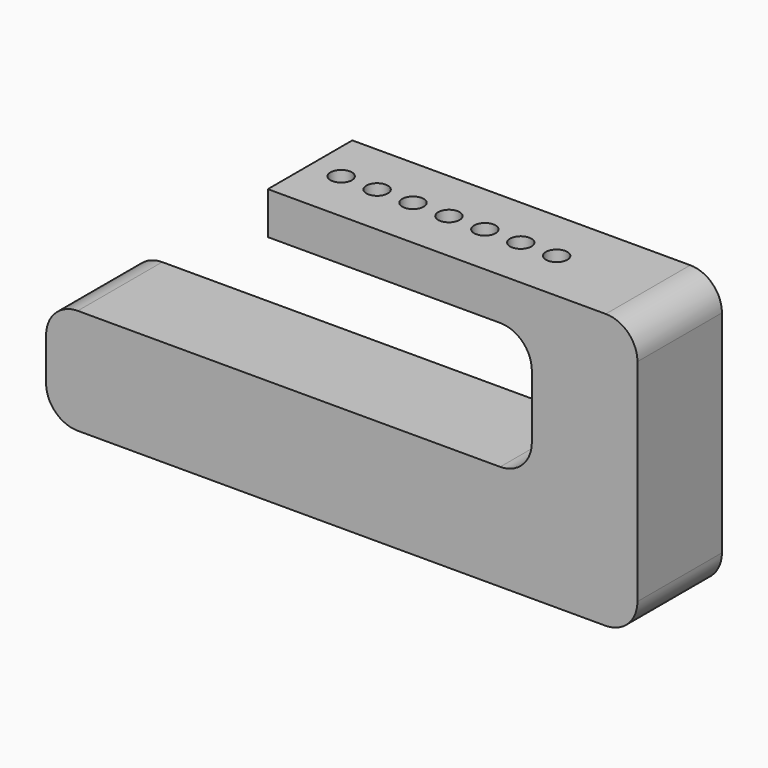
from build123d import *

# Parameters (mm, degrees)
F0_W         = 56
F0_H         = 10
F1_DEPTH     = 1.8
F2_R         = 3
F3_DEPTH     = 10
F4_W         = 10
F4_H         = 10
F5_DEPTH     = 16
F6_W         = 10
F6_H         = 4
F7_DEPTH     = 25
F8_R         = 1.0135034558
F9_DEPTH     = 10
F10_T1_DEPTH = 10
F10_T6_DEPTH = 10
F10_S7_R     = 1.0135034558
F10_T8_DEPTH = 7
F10_T9_DEPTH = 25


# Not quite as in the source:
# - a fillet or chamfer that OpenCascade refuses, or shapes differently, is made with other operations: its cross-section is extruded or revolved along the edge and cut away or added


with BuildPart() as f1:
    # F0 (on Top) → F1 (new body)
    with BuildSketch(Plane.XY):
        Rectangle(F0_W, F0_H)
    extrude(amount=F1_DEPTH)

    # F2
    f2_edges = [f1.edges().sort_by_distance(p)[0] for p in [
        (-28, 5, 0.9),
        (28, 5, 0.9),
        (28, -5, 0.9),
        (-28, -5, 0.9),
    ]]
    fillet(f2_edges, radius=F2_R)

    # F0 (on Top) → F3 (join)
    with BuildSketch(Plane.XY):
        Rectangle(F0_W, F0_H)
    extrude(amount=F3_DEPTH)

    # F4 (on face) → F5 (join)
    with BuildSketch(Plane.XY.offset(10)):
        with Locations((23, 0)):
            Rectangle(F4_W, F4_H)
    extrude(amount=F5_DEPTH)

    # F6 (on face) → F7 (join)
    with BuildSketch(Plane(origin=(18, 0, 0), x_dir=(0, -1, 0), z_dir=(-1, 0, 0))):
        with Locations((0, 24)):
            Rectangle(F6_W, F6_H)
    extrude(amount=F7_DEPTH)

    # F8 (on face) → F9 (cut)
    with BuildSketch(Plane.XY.offset(26)):
        with Locations((-4.0517724119, 0)):
            Circle(F8_R)
        with Locations((-0.6517724119, 0)):
            Circle(F8_R)
        with Locations((2.7482275881, 0)):
            Circle(F8_R)
        with Locations((6.1482275881, 0)):
            Circle(F8_R)
        with Locations((9.5482275881, 0)):
            Circle(F8_R)
        with Locations((12.9482275881, 0)):
            Circle(F8_R)
        with Locations((16.3482275881, 0)):
            Circle(F8_R)
    extrude(amount=-F9_DEPTH, mode=Mode.SUBTRACT)

    # F10: fillet of radius 3 on 6 edges, made by hand

    # F10_s2 → F10_t1 (join)
    with BuildSketch(Plane.XZ.offset(-5)):
        with BuildLine():
            ThreePointArc((18, 13), (17.1213203436, 10.8786796564), (15, 10))
            Line((15, 10), (18, 10))
            Line((18, 10), (18, 13))
        make_face()
    extrude(amount=F10_T1_DEPTH)


with BuildPart() as f10_tool4:
    # F10_s5 → F10_t6 (new body)
    with BuildSketch(Plane.XZ.offset(-5)):
        with BuildLine():
            ThreePointArc((15, 22), (17.1213203436, 21.1213203436), (18, 19))
            Line((18, 19), (18, 22))
            Line((18, 22), (15, 22))
        make_face()
    extrude(amount=F10_T6_DEPTH)

    # F10_s7 → F10_t8 (cut, symmetric)
    with BuildSketch(Plane.XY.offset(20.5)):
        with Locations((16.3482275881, 0)):
            Circle(F10_S7_R)
    extrude(amount=F10_T8_DEPTH, both=True, mode=Mode.SUBTRACT)


with BuildPart() as f1_1:
    add(f1.part)

    # F10_t3: union F10_tool4
    add(f10_tool4.part)

    # F10_s10 → F10_t9 (cut)
    with BuildSketch(Plane.XZ.offset(-12.5)):
        with BuildLine():
            ThreePointArc((25, 26), (27.1213203436, 25.1213203436), (28, 23))
            Line((28, 23), (28, 26))
            Line((28, 26), (25, 26))
        make_face()
        with BuildLine():
            ThreePointArc((28, 3), (27.1213203436, 0.8786796564), (25, 0))
            Line((25, 0), (28, 0))
            Line((28, 0), (28, 3))
        make_face()
        with BuildLine():
            ThreePointArc((-28, 3), (-27.1213203436, 0.8786796564), (-25, 0))
            Line((-25, 0), (-28, 0))
            Line((-28, 0), (-28, 3))
        make_face()
        with BuildLine():
            ThreePointArc((-28, 7), (-27.1213203436, 9.1213203436), (-25, 10))
            Line((-25, 10), (-28, 10))
            Line((-28, 10), (-28, 7))
        make_face()
    extrude(amount=F10_T9_DEPTH, mode=Mode.SUBTRACT)


solid = f1_1.part
